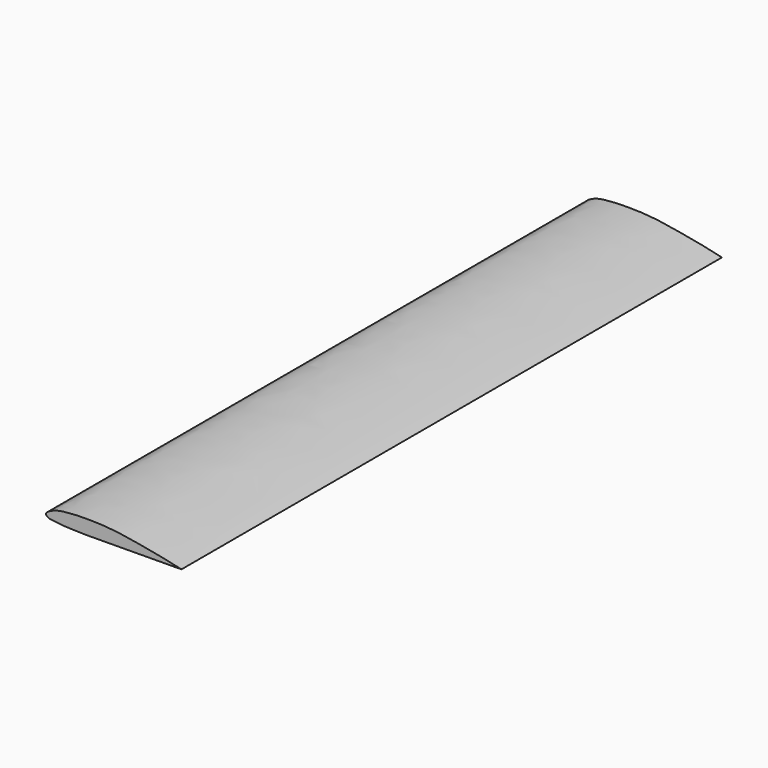
from build123d import *

# Parameters (mm, degrees)
F1_DEPTH = 1000


# Not quite as in the source:
# - a feature names something its author has since deleted; it is built from what else it names


with BuildPart() as f1:
    # F0 (on Front) → F1 (new body)
    with BuildSketch(Plane.XZ):
        with BuildLine():
            add(Edge.make_bspline(
                [(-124.0655580718, -4.386721941), (-123.3044370948, -3.6845833268), (-122.0950517914, -2.1492476316), (-116.7058944545, 0.8533666692), (-109.8761998426, 3.6737563859), (-99.6571191723, 5.8254945739), (-86.6767282827, 6.7198393742), (-76.3816754653, 7.6349539484), (-52.2756101525, 7.4535026051), (-42.7616771756, 7.1169717413), (-28.5458332747, 6.0155421708), (-13.2661231215, 4.6025471767), (13.575560063, -0.1789631068), (38.5797105731, -4.4574796256), (60.0739421044, -9.0349682194), (71.0236573709, -11.5474682288), (76.1711355444, -12.7252812378)],
                knots=[0, 0, 0, 0, 0.033100321, 0.0798604167, 0.1328430623, 0.195700391, 0.2642812543, 0.3289957623, 0.4226325294, 0.4846008011, 0.5549534026, 0.6316604189, 0.732473743, 0.8317483554, 0.9219346899, 1, 1, 1, 1], degree=3))
            Line((-124.0655580718, -4.386721941), (-124.2522768608, -6.6810622362))
            add(Edge.make_bspline(
                [(-124.2522768608, -6.6810622362), (-123.8288644556, -7.2320381285), (-122.8536975345, -8.5009984338), (-119.684022261, -10.6586279453), (-112.6366169608, -11.3396613327), (-107.2981776041, -12.0631029916), (-94.2335164877, -13.0906799487), (-84.1420398981, -13.1958665568), (-72.0937462666, -13.5664284327), (-65.1942115304, -13.7786334446)],
                knots=[0, 0, 0, 0, 0.0754442327, 0.1737566683, 0.3069425072, 0.4297933177, 0.6104875682, 0.7769431082, 1, 1, 1, 1], degree=3))
            Line((-65.1942115304, -13.7786334446), (76.1711355444, -12.7252812378))
        make_face()
    extrude(amount=F1_DEPTH)


solid = f1.part
